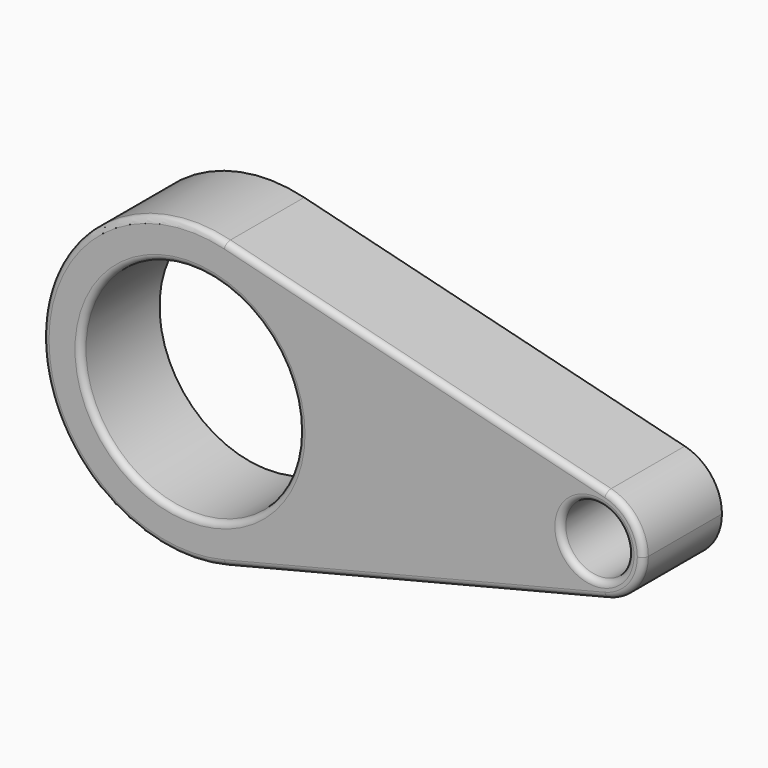
from build123d import *

# Parameters (mm, degrees)
F1_DEPTH = 50.8
F2_R     = 56.411599825
F2_R_2   = 17.3341868335
F3_DEPTH = 50.8
F4_R     = 3.175
F5_T     = -2.54


with BuildPart() as f1:
    # F0 (on Front) → F1 (new body)
    with BuildSketch(Plane.XZ):
        with BuildLine():
            ThreePointArc((18.4812146278, 73.9248585111), (60.0612543768, 46.8944103565), (76.2, 0))
            ThreePointArc((76.2, 0), (60.0612543768, -46.8944103565), (18.4812146278, -73.9248585111))
            Line((18.4812146278, -73.9248585111), (215.6141706573, -24.6416195037))
            ThreePointArc((215.6141706573, -24.6416195037), (184.0537657814, 0), (215.6141706573, 24.6416195037))
            Line((215.6141706573, 24.6416195037), (18.4812146278, 73.9248585111))
        make_face()
        with BuildLine():
            ThreePointArc((234.8537657814, 0), (229.474183907, 15.6314701188), (215.6141706573, 24.6416195037))
            ThreePointArc((215.6141706573, 24.6416195037), (184.0537657814, 0), (215.6141706573, -24.6416195037))
            ThreePointArc((215.6141706573, -24.6416195037), (229.474183907, -15.6314701188), (234.8537657814, 0))
        make_face()
        with BuildLine():
            ThreePointArc((18.4812146278, -73.9248585111), (60.0612543768, -46.8944103565), (76.2, 0))
            ThreePointArc((76.2, 0), (60.0612543768, 46.8944103565), (18.4812146278, 73.9248585111))
            ThreePointArc((18.4812146278, 73.9248585111), (-76.2, 0), (18.4812146278, -73.9248585111))
        make_face()
    extrude(amount=F1_DEPTH)

    # F2 (on face) → F3 (cut)
    with BuildSketch(Plane.XZ.offset(50.8)):
        Circle(F2_R)
        with Locations((209.4537657814, 0)):
            Circle(F2_R_2)
    extrude(amount=-F3_DEPTH, mode=Mode.SUBTRACT)

    # F4
    f4_edges = [f1.edges().sort_by_distance(p)[0] for p in [
        (117.047693, -50.8, 49.283239),
        (234.853766, -50.8, 0),
        (-76.2, -50.8, 0),
        (117.047693, -50.8, -49.283239),
        (-56.4116, -50.8, 0),
        (192.119579, -50.8, 0),
    ]]
    fillet(f4_edges, radius=F4_R)

    # F5
    f5_openings = [f1.faces().sort_by_distance(p)[0] for p in [
        (77.972977, 0, 0),
    ]]
    offset(amount=F5_T, openings=f5_openings)


solid = f1.part
